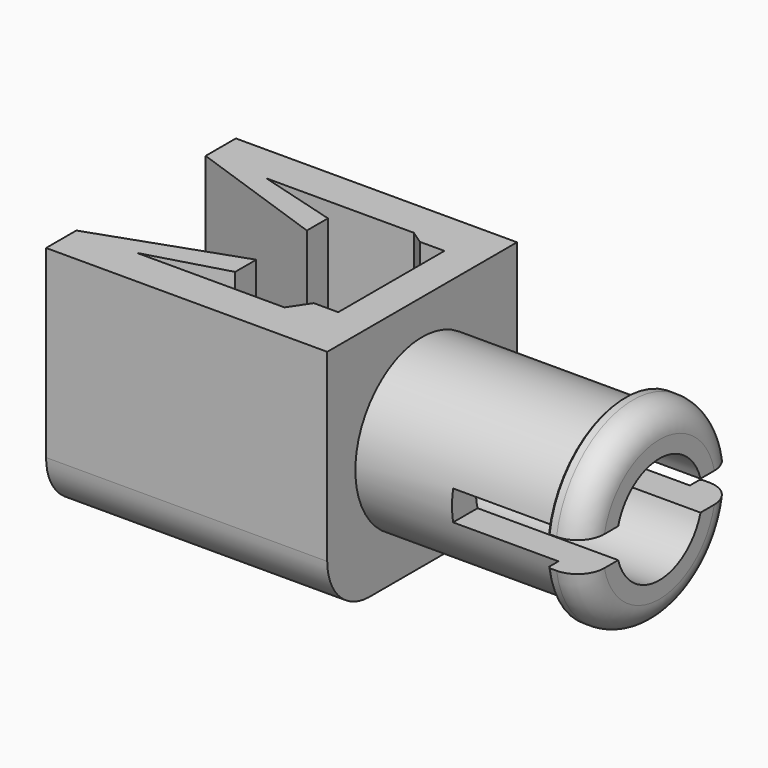
from build123d import *

# Parameters (mm, degrees)
F0_W          = 16
F0_H          = 13.5
F1_DEPTH      = 13.5
F2_R          = 4.75
F3_DEPTH      = 11.5
F4_R          = 5.5
F5_DEPTH      = 2
F7_DEPTH      = 11
F8_R          = 3.05
F9_DEPTH      = 17
F10_W         = 9.2
F10_H         = 2.4967868254
F11_DEPTH     = 10
F12_W         = 12.1366479748
F12_H         = 1.7
F13_DEPTH     = 8
F14_T4_DEPTH  = 19.347977845
F14_T9_DEPTH  = 19.347977845
F14_T11_DEPTH = 31
F15_R         = 1.5
F16_SIZE      = 0.1


# Not quite as in the source:
# - a fillet or chamfer that OpenCascade refuses, or shapes differently, is made with other operations: its cross-section is extruded or revolved along the edge and cut away or added


with BuildPart() as f1:
    # F0 (on Top) → F1 (new body)
    with BuildSketch(Plane.XY):
        Rectangle(F0_W, F0_H)
    extrude(amount=F1_DEPTH)

    # F2 (on face) → F3 (join)
    with BuildSketch(Plane.YZ.offset(8)):
        with Locations((0, 6.75)):
            Circle(F2_R)
    extrude(amount=F3_DEPTH)

    # F4 (on face) → F5 (join)
    with BuildSketch(Plane.YZ.offset(19.5)):
        with Locations((0, 6.75)):
            Circle(F4_R)
    extrude(amount=F5_DEPTH)

    # F6 (on face) → F7 (cut)
    with BuildSketch(Plane.XY.offset(13.5)):
        Polygon((0, 3.3), (0, 1.8), (-8, 4.6), (-8, -4.6), (0, -1.8), (0, -3.3), (-4.5499948867, -4.6), (3.847977845, -4.6), (4.6067554504, -3.4655697951), (6, -3.4655697951), (6, 4.0877170554), (4.6067554504, 4.0877170554), (3.847977845, 4.6), (-4.5499948867, 4.6), align=None)
    extrude(amount=-F7_DEPTH, mode=Mode.SUBTRACT)

    # F8 (on face) → F9 (cut)
    with BuildSketch(Plane.YZ.offset(21.5)):
        with Locations((0, 6.75)):
            Circle(F8_R)
    extrude(amount=-F9_DEPTH, mode=Mode.SUBTRACT)

    # F10 (on face) → F11 (cut)
    with BuildSketch(Plane(origin=(-8, 0, 0), x_dir=(0, -1, 0), z_dir=(-1, 0, 0))):
        with Locations((0, 3.7483934127)):
            Rectangle(F10_W, F10_H)
    extrude(amount=-F11_DEPTH, mode=Mode.SUBTRACT)

    # F12 (on face) → F13 (cut)
    with BuildSketch(Plane.YZ.offset(21.5)):
        with Locations((0, 6.75)):
            Rectangle(F12_W, F12_H)
    extrude(amount=-F13_DEPTH, mode=Mode.SUBTRACT)

    # F14: fillet of radius 3 on 4 edges, made by hand


with BuildPart() as f14_tool2:
    # F14_s3 → F14_t4 (new body)
    with BuildSketch(Plane.YZ.offset(11.347977845)):
        with BuildLine():
            ThreePointArc((1.6, 2.5), (3.7213203436, 3.3786796564), (4.6, 5.5))
            Line((4.6, 5.5), (4.6, 2.5))
            Line((4.6, 2.5), (1.6, 2.5))
        make_face()
    extrude(amount=-F14_T4_DEPTH)

    split(bisect_by=Plane.YZ.offset(6), keep=Keep.BOTTOM)


with BuildPart() as f1_1:
    add(f1.part)

    # F14_t1: union F14_tool2
    add(f14_tool2.part)


with BuildPart() as f14_tool7:
    # F14_s8 → F14_t9 (new body)
    with BuildSketch(Plane.YZ.offset(-8)):
        with BuildLine():
            ThreePointArc((-1.6, 2.5), (-3.7213203436, 3.3786796564), (-4.6, 5.5))
            Line((-4.6, 5.5), (-4.6, 2.5))
            Line((-4.6, 2.5), (-1.6, 2.5))
        make_face()
    extrude(amount=F14_T9_DEPTH)

    split(bisect_by=Plane.YZ.offset(6), keep=Keep.BOTTOM)


with BuildPart() as f1_2:
    add(f1_1.part)

    # F14_t6: union F14_tool7
    add(f14_tool7.part)

    # F14_s12 → F14_t11 (cut)
    with BuildSketch(Plane.YZ.offset(-15.5)):
        with BuildLine():
            ThreePointArc((3.75, 0), (5.8713203436, 0.8786796564), (6.75, 3))
            Line((6.75, 3), (6.75, 0))
            Line((6.75, 0), (3.75, 0))
        make_face()
        with BuildLine():
            ThreePointArc((-6.75, 3), (-5.8713203436, 0.8786796564), (-3.75, 0))
            Line((-3.75, 0), (-6.75, 0))
            Line((-6.75, 0), (-6.75, 3))
        make_face()
    extrude(amount=F14_T11_DEPTH, mode=Mode.SUBTRACT)

    # F15
    f15_edges = [f1_2.edges().sort_by_distance(p)[0] for p in [
        (21.5, 0, 12.25),
        (21.5, 0, 1.25),
    ]]
    fillet(f15_edges, radius=F15_R)

    # F16
    f16_edges = [f1_2.edges().sort_by_distance(p)[0] for p in [
        (19.5, 0, 1.25),
        (19.5, 0, 12.25),
    ]]
    chamfer(f16_edges, length=F16_SIZE)


solid = f1_2.part
